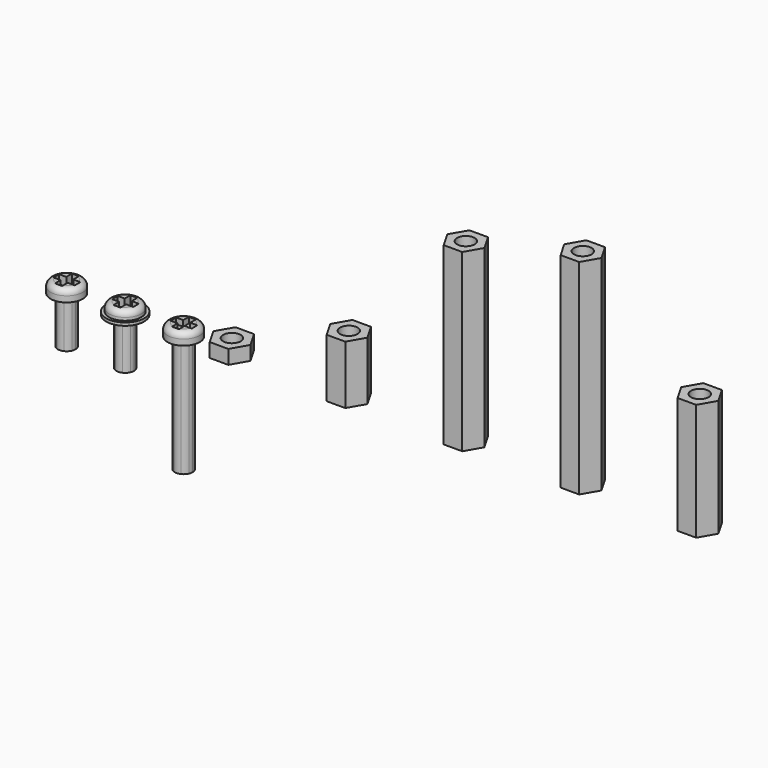
from build123d import *

# Parameters (mm, degrees)
F0_R      = 1.5
F1_DEPTH  = 2.4
F2_DEPTH  = 10
F3_DEPTH  = 30
F4_R      = 2.75
F5_DEPTH  = 2
F6_DEPTH  = 2
F7_DEPTH  = 0.5
F8_DEPTH  = 8
F4_R_2    = 3.25
F12_DEPTH = 0.5
F14_DEPTH = 35
F16_DEPTH = 20
F19_DEPTH = 2
F20_DEPTH = 2
F21_DEPTH = 1
F22_DEPTH = 20


# Not quite as in the source:
# - a fillet or chamfer that OpenCascade refuses, or shapes differently, is made with other operations: its cross-section is extruded or revolved along the edge and cut away or added


with BuildPart() as f1:
    # F0 (on Top) → F1 (new body)
    with BuildSketch(Plane.XY):
        Polygon((1.5877132403, -2.75), (3.1754264805, 0), (1.5877132403, 2.75), (-1.5877132403, 2.75), (-3.1754264805, 0), (-1.5877132403, -2.75), align=None)
        Circle(F0_R, mode=Mode.SUBTRACT)
    extrude(amount=F1_DEPTH)


with BuildPart() as f2:
    # F0 (on Top) → F2 (new body)
    with BuildSketch(Plane.XY):
        Polygon((1.5877132403, -2.75), (3.1754264805, 0), (1.5877132403, 2.75), (-1.5877132403, 2.75), (-3.1754264805, 0), (-1.5877132403, -2.75), align=None)
        Circle(F0_R, mode=Mode.SUBTRACT)
    extrude(amount=F2_DEPTH)


with BuildPart() as f3:
    # F0 (on Top) → F3 (new body)
    with BuildSketch(Plane.XY):
        Polygon((1.5877132403, -2.75), (3.1754264805, 0), (1.5877132403, 2.75), (-1.5877132403, 2.75), (-3.1754264805, 0), (-1.5877132403, -2.75), align=None)
        Circle(F0_R, mode=Mode.SUBTRACT)
    extrude(amount=F3_DEPTH)


with BuildPart() as f5:
    # F4 (on Top) → F5 (new body)
    with BuildSketch(Plane.XY):
        with Locations((-8.2484744489, 0)):
            Circle(F4_R)
        with BuildLine():
            ThreePointArc((-7.6, 1.3525830433), (-7.1691331802, 1.0416440974), (-6.8737017404, 0.6))
            Line((-6.8737017404, 0.6), (-6.4, 0.6))
            Line((-6.4, 0.6), (-6.4, -0.6))
            Line((-6.4, -0.6), (-6.8737017404, -0.6))
            ThreePointArc((-6.8737017404, -0.6), (-7.1691331802, -1.0416440974), (-7.6, -1.3525830433))
            Line((-7.6, -1.3525830433), (-7.6, -1.8))
            Line((-7.6, -1.8), (-8.8, -1.8))
            Line((-8.8, -1.8), (-8.8, -1.394926366))
            ThreePointArc((-8.8, -1.394926366), (-9.2904116966, -1.0790582802), (-9.6232471574, -0.6))
            Line((-9.6232471574, -0.6), (-10, -0.6))
            Line((-10, -0.6), (-10, 0.6))
            Line((-10, 0.6), (-9.6232471574, 0.6))
            ThreePointArc((-9.6232471574, 0.6), (-9.2904116966, 1.0790582802), (-8.8, 1.394926366))
            Line((-8.8, 1.394926366), (-8.8, 1.8))
            Line((-8.8, 1.8), (-7.6, 1.8))
            Line((-7.6, 1.8), (-7.6, 1.3525830433))
        make_face(mode=Mode.SUBTRACT)
        with BuildLine():
            ThreePointArc((-9.6232471574, -0.6), (-9.2904116966, -1.0790582802), (-8.8, -1.394926366))
            Line((-8.8, -1.394926366), (-8.8, -0.6))
            Line((-8.8, -0.6), (-9.6232471574, -0.6))
        make_face()
        with BuildLine():
            ThreePointArc((-9.6232471574, -0.6), (-9.7484744489, 0), (-9.6232471574, 0.6))
            Line((-9.6232471574, 0.6), (-10, 0.6))
            Line((-10, 0.6), (-10, -0.6))
            Line((-10, -0.6), (-9.6232471574, -0.6))
        make_face()
        with BuildLine():
            Line((-7.6, -1.8), (-7.6, -1.3525830433))
            ThreePointArc((-7.6, -1.3525830433), (-8.1955782161, -1.4990670394), (-8.8, -1.394926366))
            Line((-8.8, -1.394926366), (-8.8, -1.8))
            Line((-8.8, -1.8), (-7.6, -1.8))
        make_face()
        with BuildLine():
            ThreePointArc((-7.6, -1.3525830433), (-7.1691331802, -1.0416440974), (-6.8737017404, -0.6))
            Line((-6.8737017404, -0.6), (-7.6, -0.6))
            Line((-7.6, -0.6), (-7.6, -1.3525830433))
        make_face()
        with BuildLine():
            ThreePointArc((-6.8737017404, 0.6), (-6.7801149795, 0.3064644655), (-6.7484744489, 0))
            ThreePointArc((-6.7484744489, 0), (-6.7801149795, -0.3064644655), (-6.8737017404, -0.6))
            Line((-6.8737017404, -0.6), (-6.4, -0.6))
            Line((-6.4, -0.6), (-6.4, 0.6))
            Line((-6.4, 0.6), (-6.8737017404, 0.6))
        make_face()
        with BuildLine():
            Line((-7.6, 0.6), (-6.8737017404, 0.6))
            ThreePointArc((-6.8737017404, 0.6), (-7.1691331802, 1.0416440974), (-7.6, 1.3525830433))
            Line((-7.6, 1.3525830433), (-7.6, 0.6))
        make_face()
        with BuildLine():
            ThreePointArc((-8.8, 1.394926366), (-8.1955782161, 1.4990670394), (-7.6, 1.3525830433))
            Line((-7.6, 1.3525830433), (-7.6, 1.8))
            Line((-7.6, 1.8), (-8.8, 1.8))
            Line((-8.8, 1.8), (-8.8, 1.394926366))
        make_face()
        with BuildLine():
            Line((-8.8, 0.6), (-8.8, 1.394926366))
            ThreePointArc((-8.8, 1.394926366), (-9.2904116966, 1.0790582802), (-9.6232471574, 0.6))
            Line((-9.6232471574, 0.6), (-8.8, 0.6))
        make_face()
        with BuildLine():
            ThreePointArc((-6.8737017404, -0.6), (-6.7801149795, -0.3064644655), (-6.7484744489, 0))
            ThreePointArc((-6.7484744489, 0), (-6.7801149795, 0.3064644655), (-6.8737017404, 0.6))
            Line((-6.8737017404, 0.6), (-7.6, 0.6))
            Line((-7.6, 0.6), (-7.6, 1.3525830433))
            ThreePointArc((-7.6, 1.3525830433), (-8.1955782161, 1.4990670394), (-8.8, 1.394926366))
            Line((-8.8, 1.394926366), (-8.8, 0.6))
            Line((-8.8, 0.6), (-9.6232471574, 0.6))
            ThreePointArc((-9.6232471574, 0.6), (-9.7484744489, 0), (-9.6232471574, -0.6))
            Line((-9.6232471574, -0.6), (-8.8, -0.6))
            Line((-8.8, -0.6), (-8.8, -1.394926366))
            ThreePointArc((-8.8, -1.394926366), (-8.1955782161, -1.4990670394), (-7.6, -1.3525830433))
            Line((-7.6, -1.3525830433), (-7.6, -0.6))
            Line((-7.6, -0.6), (-6.8737017404, -0.6))
        make_face()
    extrude(amount=F5_DEPTH)

    # F4 (on Top) → F6 (cut)
    with BuildSketch(Plane.XY):
        with BuildLine():
            ThreePointArc((-9.6232471574, -0.6), (-9.7484744489, 0), (-9.6232471574, 0.6))
            Line((-9.6232471574, 0.6), (-10, 0.6))
            Line((-10, 0.6), (-10, -0.6))
            Line((-10, -0.6), (-9.6232471574, -0.6))
        make_face()
        with BuildLine():
            ThreePointArc((-6.8737017404, -0.6), (-6.7801149795, -0.3064644655), (-6.7484744489, 0))
            ThreePointArc((-6.7484744489, 0), (-6.7801149795, 0.3064644655), (-6.8737017404, 0.6))
            Line((-6.8737017404, 0.6), (-7.6, 0.6))
            Line((-7.6, 0.6), (-7.6, 1.3525830433))
            ThreePointArc((-7.6, 1.3525830433), (-8.1955782161, 1.4990670394), (-8.8, 1.394926366))
            Line((-8.8, 1.394926366), (-8.8, 0.6))
            Line((-8.8, 0.6), (-9.6232471574, 0.6))
            ThreePointArc((-9.6232471574, 0.6), (-9.7484744489, 0), (-9.6232471574, -0.6))
            Line((-9.6232471574, -0.6), (-8.8, -0.6))
            Line((-8.8, -0.6), (-8.8, -1.394926366))
            ThreePointArc((-8.8, -1.394926366), (-8.1955782161, -1.4990670394), (-7.6, -1.3525830433))
            Line((-7.6, -1.3525830433), (-7.6, -0.6))
            Line((-7.6, -0.6), (-6.8737017404, -0.6))
        make_face()
        with BuildLine():
            ThreePointArc((-6.8737017404, 0.6), (-6.7801149795, 0.3064644655), (-6.7484744489, 0))
            ThreePointArc((-6.7484744489, 0), (-6.7801149795, -0.3064644655), (-6.8737017404, -0.6))
            Line((-6.8737017404, -0.6), (-6.4, -0.6))
            Line((-6.4, -0.6), (-6.4, 0.6))
            Line((-6.4, 0.6), (-6.8737017404, 0.6))
        make_face()
        with BuildLine():
            Line((-7.6, -1.8), (-7.6, -1.3525830433))
            ThreePointArc((-7.6, -1.3525830433), (-8.1955782161, -1.4990670394), (-8.8, -1.394926366))
            Line((-8.8, -1.394926366), (-8.8, -1.8))
            Line((-8.8, -1.8), (-7.6, -1.8))
        make_face()
        with BuildLine():
            ThreePointArc((-8.8, 1.394926366), (-8.1955782161, 1.4990670394), (-7.6, 1.3525830433))
            Line((-7.6, 1.3525830433), (-7.6, 1.8))
            Line((-7.6, 1.8), (-8.8, 1.8))
            Line((-8.8, 1.8), (-8.8, 1.394926366))
        make_face()
    extrude(amount=F6_DEPTH, mode=Mode.SUBTRACT)

    # F4 (on Top) → F7 (join)
    with BuildSketch(Plane.XY):
        with Locations((-8.2484744489, 0)):
            Circle(F4_R)
        with BuildLine():
            ThreePointArc((-7.6, 1.3525830433), (-7.1691331802, 1.0416440974), (-6.8737017404, 0.6))
            Line((-6.8737017404, 0.6), (-6.4, 0.6))
            Line((-6.4, 0.6), (-6.4, -0.6))
            Line((-6.4, -0.6), (-6.8737017404, -0.6))
            ThreePointArc((-6.8737017404, -0.6), (-7.1691331802, -1.0416440974), (-7.6, -1.3525830433))
            Line((-7.6, -1.3525830433), (-7.6, -1.8))
            Line((-7.6, -1.8), (-8.8, -1.8))
            Line((-8.8, -1.8), (-8.8, -1.394926366))
            ThreePointArc((-8.8, -1.394926366), (-9.2904116966, -1.0790582802), (-9.6232471574, -0.6))
            Line((-9.6232471574, -0.6), (-10, -0.6))
            Line((-10, -0.6), (-10, 0.6))
            Line((-10, 0.6), (-9.6232471574, 0.6))
            ThreePointArc((-9.6232471574, 0.6), (-9.2904116966, 1.0790582802), (-8.8, 1.394926366))
            Line((-8.8, 1.394926366), (-8.8, 1.8))
            Line((-8.8, 1.8), (-7.6, 1.8))
            Line((-7.6, 1.8), (-7.6, 1.3525830433))
        make_face(mode=Mode.SUBTRACT)
        with BuildLine():
            ThreePointArc((-9.6232471574, -0.6), (-9.2904116966, -1.0790582802), (-8.8, -1.394926366))
            Line((-8.8, -1.394926366), (-8.8, -0.6))
            Line((-8.8, -0.6), (-9.6232471574, -0.6))
        make_face()
        with BuildLine():
            Line((-7.6, -1.8), (-7.6, -1.3525830433))
            ThreePointArc((-7.6, -1.3525830433), (-8.1955782161, -1.4990670394), (-8.8, -1.394926366))
            Line((-8.8, -1.394926366), (-8.8, -1.8))
            Line((-8.8, -1.8), (-7.6, -1.8))
        make_face()
        with BuildLine():
            ThreePointArc((-7.6, -1.3525830433), (-7.1691331802, -1.0416440974), (-6.8737017404, -0.6))
            Line((-6.8737017404, -0.6), (-7.6, -0.6))
            Line((-7.6, -0.6), (-7.6, -1.3525830433))
        make_face()
        with BuildLine():
            ThreePointArc((-6.8737017404, 0.6), (-6.7801149795, 0.3064644655), (-6.7484744489, 0))
            ThreePointArc((-6.7484744489, 0), (-6.7801149795, -0.3064644655), (-6.8737017404, -0.6))
            Line((-6.8737017404, -0.6), (-6.4, -0.6))
            Line((-6.4, -0.6), (-6.4, 0.6))
            Line((-6.4, 0.6), (-6.8737017404, 0.6))
        make_face()
        with BuildLine():
            ThreePointArc((-6.8737017404, -0.6), (-6.7801149795, -0.3064644655), (-6.7484744489, 0))
            ThreePointArc((-6.7484744489, 0), (-6.7801149795, 0.3064644655), (-6.8737017404, 0.6))
            Line((-6.8737017404, 0.6), (-7.6, 0.6))
            Line((-7.6, 0.6), (-7.6, 1.3525830433))
            ThreePointArc((-7.6, 1.3525830433), (-8.1955782161, 1.4990670394), (-8.8, 1.394926366))
            Line((-8.8, 1.394926366), (-8.8, 0.6))
            Line((-8.8, 0.6), (-9.6232471574, 0.6))
            ThreePointArc((-9.6232471574, 0.6), (-9.7484744489, 0), (-9.6232471574, -0.6))
            Line((-9.6232471574, -0.6), (-8.8, -0.6))
            Line((-8.8, -0.6), (-8.8, -1.394926366))
            ThreePointArc((-8.8, -1.394926366), (-8.1955782161, -1.4990670394), (-7.6, -1.3525830433))
            Line((-7.6, -1.3525830433), (-7.6, -0.6))
            Line((-7.6, -0.6), (-6.8737017404, -0.6))
        make_face()
        with BuildLine():
            ThreePointArc((-8.8, 1.394926366), (-8.1955782161, 1.4990670394), (-7.6, 1.3525830433))
            Line((-7.6, 1.3525830433), (-7.6, 1.8))
            Line((-7.6, 1.8), (-8.8, 1.8))
            Line((-8.8, 1.8), (-8.8, 1.394926366))
        make_face()
        with BuildLine():
            Line((-8.8, 0.6), (-8.8, 1.394926366))
            ThreePointArc((-8.8, 1.394926366), (-9.2904116966, 1.0790582802), (-9.6232471574, 0.6))
            Line((-9.6232471574, 0.6), (-8.8, 0.6))
        make_face()
        with BuildLine():
            Line((-7.6, 0.6), (-6.8737017404, 0.6))
            ThreePointArc((-6.8737017404, 0.6), (-7.1691331802, 1.0416440974), (-7.6, 1.3525830433))
            Line((-7.6, 1.3525830433), (-7.6, 0.6))
        make_face()
        with BuildLine():
            ThreePointArc((-9.6232471574, -0.6), (-9.7484744489, 0), (-9.6232471574, 0.6))
            Line((-9.6232471574, 0.6), (-10, 0.6))
            Line((-10, 0.6), (-10, -0.6))
            Line((-10, -0.6), (-9.6232471574, -0.6))
        make_face()
    extrude(amount=F7_DEPTH)

    # F4 (on Top) → F8 (join)
    with BuildSketch(Plane.XY):
        with BuildLine():
            ThreePointArc((-9.6232471574, -0.6), (-9.2904116966, -1.0790582802), (-8.8, -1.394926366))
            Line((-8.8, -1.394926366), (-8.8, -0.6))
            Line((-8.8, -0.6), (-9.6232471574, -0.6))
        make_face()
        with BuildLine():
            ThreePointArc((-6.8737017404, -0.6), (-6.7801149795, -0.3064644655), (-6.7484744489, 0))
            ThreePointArc((-6.7484744489, 0), (-6.7801149795, 0.3064644655), (-6.8737017404, 0.6))
            Line((-6.8737017404, 0.6), (-7.6, 0.6))
            Line((-7.6, 0.6), (-7.6, 1.3525830433))
            ThreePointArc((-7.6, 1.3525830433), (-8.1955782161, 1.4990670394), (-8.8, 1.394926366))
            Line((-8.8, 1.394926366), (-8.8, 0.6))
            Line((-8.8, 0.6), (-9.6232471574, 0.6))
            ThreePointArc((-9.6232471574, 0.6), (-9.7484744489, 0), (-9.6232471574, -0.6))
            Line((-9.6232471574, -0.6), (-8.8, -0.6))
            Line((-8.8, -0.6), (-8.8, -1.394926366))
            ThreePointArc((-8.8, -1.394926366), (-8.1955782161, -1.4990670394), (-7.6, -1.3525830433))
            Line((-7.6, -1.3525830433), (-7.6, -0.6))
            Line((-7.6, -0.6), (-6.8737017404, -0.6))
        make_face()
        with BuildLine():
            ThreePointArc((-7.6, -1.3525830433), (-7.1691331802, -1.0416440974), (-6.8737017404, -0.6))
            Line((-6.8737017404, -0.6), (-7.6, -0.6))
            Line((-7.6, -0.6), (-7.6, -1.3525830433))
        make_face()
        with BuildLine():
            Line((-8.8, 0.6), (-8.8, 1.394926366))
            ThreePointArc((-8.8, 1.394926366), (-9.2904116966, 1.0790582802), (-9.6232471574, 0.6))
            Line((-9.6232471574, 0.6), (-8.8, 0.6))
        make_face()
        with BuildLine():
            Line((-7.6, 0.6), (-6.8737017404, 0.6))
            ThreePointArc((-6.8737017404, 0.6), (-7.1691331802, 1.0416440974), (-7.6, 1.3525830433))
            Line((-7.6, 1.3525830433), (-7.6, 0.6))
        make_face()
    extrude(amount=-F8_DEPTH)


with BuildPart() as f2_1:
    # F9: moved
    add(f2.part.moved(Location((20, 0, 0))))


with BuildPart() as f3_1:
    # F10: moved
    add(f3.part.moved(Location((40, 0, 0))))


with BuildPart() as f11_1:
    # F11: copy of F5
    add(f5.part.moved(Location((-20, 0, 0))))

    # F13: fillet of radius 1 on 1 edges, made by hand

    # F13_s1 → F13_t2 (revolve, cut)
    with BuildSketch(Plane.XZ):
        with BuildLine():
            ThreePointArc((-25.4984744489, 1), (-25.7913676677, 1.7071067812), (-26.4984744489, 2))
            Line((-26.4984744489, 2), (-25.4984744489, 2))
            Line((-25.4984744489, 2), (-25.4984744489, 1))
        make_face()
    revolve(axis=Axis((-28.2484744489, 0, 2), (0, 0, 1)), mode=Mode.SUBTRACT)


with BuildPart() as f5_1:
    add(f5.part)

    # F4 (on Top) → F12 (join)
    with BuildSketch(Plane.XY):
        with Locations((-8.2484744489, 0)):
            Circle(F4_R_2)
        with Locations((-8.2484744489, 0)):
            Circle(F4_R, mode=Mode.SUBTRACT)
    extrude(amount=F12_DEPTH)

    # F13#2: fillet of radius 1 on 1 edges, made by hand

    # F13_2_s1 → F13_2_t2 (revolve, cut)
    with BuildSketch(Plane.XZ):
        with BuildLine():
            ThreePointArc((-5.4984744489, 1), (-5.7913676677, 1.7071067812), (-6.4984744489, 2))
            Line((-6.4984744489, 2), (-5.4984744489, 2))
            Line((-5.4984744489, 2), (-5.4984744489, 1))
        make_face()
    revolve(axis=Axis((-8.2484744489, 0, 2), (0, 0, 1)), mode=Mode.SUBTRACT)


with BuildPart() as f14:
    # F0 (on Top) → F14 (new body)
    with BuildSketch(Plane.XY):
        Polygon((1.5877132403, -2.75), (3.1754264805, 0), (1.5877132403, 2.75), (-1.5877132403, 2.75), (-3.1754264805, 0), (-1.5877132403, -2.75), align=None)
        Circle(F0_R, mode=Mode.SUBTRACT)
    extrude(amount=F14_DEPTH)


with BuildPart() as f14_1:
    # F15: moved
    add(f14.part.moved(Location((60, 0, 0))))


with BuildPart() as f16:
    # F0 (on Top) → F16 (new body)
    with BuildSketch(Plane.XY):
        Polygon((1.5877132403, -2.75), (3.1754264805, 0), (1.5877132403, 2.75), (-1.5877132403, 2.75), (-3.1754264805, 0), (-1.5877132403, -2.75), align=None)
        Circle(F0_R, mode=Mode.SUBTRACT)
    extrude(amount=F16_DEPTH)


with BuildPart() as f16_1:
    # F17: moved
    add(f16.part.moved(Location((80, 0, 0))))


with BuildPart() as f5_2:
    # F18: moved
    add(f5_1.part.moved(Location((-10, 0, 0))))


with BuildPart() as f19:
    # F4 (on Top) → F19 (new body)
    with BuildSketch(Plane.XY):
        with Locations((-8.2484744489, 0)):
            Circle(F4_R)
        with BuildLine():
            ThreePointArc((-7.6, 1.3525830433), (-7.1691331802, 1.0416440974), (-6.8737017404, 0.6))
            Line((-6.8737017404, 0.6), (-6.4, 0.6))
            Line((-6.4, 0.6), (-6.4, -0.6))
            Line((-6.4, -0.6), (-6.8737017404, -0.6))
            ThreePointArc((-6.8737017404, -0.6), (-7.1691331802, -1.0416440974), (-7.6, -1.3525830433))
            Line((-7.6, -1.3525830433), (-7.6, -1.8))
            Line((-7.6, -1.8), (-8.8, -1.8))
            Line((-8.8, -1.8), (-8.8, -1.394926366))
            ThreePointArc((-8.8, -1.394926366), (-9.2904116966, -1.0790582802), (-9.6232471574, -0.6))
            Line((-9.6232471574, -0.6), (-10, -0.6))
            Line((-10, -0.6), (-10, 0.6))
            Line((-10, 0.6), (-9.6232471574, 0.6))
            ThreePointArc((-9.6232471574, 0.6), (-9.2904116966, 1.0790582802), (-8.8, 1.394926366))
            Line((-8.8, 1.394926366), (-8.8, 1.8))
            Line((-8.8, 1.8), (-7.6, 1.8))
            Line((-7.6, 1.8), (-7.6, 1.3525830433))
        make_face(mode=Mode.SUBTRACT)
        with BuildLine():
            ThreePointArc((-6.8737017404, 0.6), (-6.7801149795, 0.3064644655), (-6.7484744489, 0))
            ThreePointArc((-6.7484744489, 0), (-6.7801149795, -0.3064644655), (-6.8737017404, -0.6))
            Line((-6.8737017404, -0.6), (-6.4, -0.6))
            Line((-6.4, -0.6), (-6.4, 0.6))
            Line((-6.4, 0.6), (-6.8737017404, 0.6))
        make_face()
        with BuildLine():
            ThreePointArc((-7.6, -1.3525830433), (-7.1691331802, -1.0416440974), (-6.8737017404, -0.6))
            Line((-6.8737017404, -0.6), (-7.6, -0.6))
            Line((-7.6, -0.6), (-7.6, -1.3525830433))
        make_face()
        with BuildLine():
            ThreePointArc((-9.6232471574, -0.6), (-9.2904116966, -1.0790582802), (-8.8, -1.394926366))
            Line((-8.8, -1.394926366), (-8.8, -0.6))
            Line((-8.8, -0.6), (-9.6232471574, -0.6))
        make_face()
        with BuildLine():
            Line((-7.6, -1.8), (-7.6, -1.3525830433))
            ThreePointArc((-7.6, -1.3525830433), (-8.1955782161, -1.4990670394), (-8.8, -1.394926366))
            Line((-8.8, -1.394926366), (-8.8, -1.8))
            Line((-8.8, -1.8), (-7.6, -1.8))
        make_face()
        with BuildLine():
            ThreePointArc((-9.6232471574, -0.6), (-9.7484744489, 0), (-9.6232471574, 0.6))
            Line((-9.6232471574, 0.6), (-10, 0.6))
            Line((-10, 0.6), (-10, -0.6))
            Line((-10, -0.6), (-9.6232471574, -0.6))
        make_face()
        with BuildLine():
            ThreePointArc((-8.8, 1.394926366), (-8.1955782161, 1.4990670394), (-7.6, 1.3525830433))
            Line((-7.6, 1.3525830433), (-7.6, 1.8))
            Line((-7.6, 1.8), (-8.8, 1.8))
            Line((-8.8, 1.8), (-8.8, 1.394926366))
        make_face()
        with BuildLine():
            Line((-7.6, 0.6), (-6.8737017404, 0.6))
            ThreePointArc((-6.8737017404, 0.6), (-7.1691331802, 1.0416440974), (-7.6, 1.3525830433))
            Line((-7.6, 1.3525830433), (-7.6, 0.6))
        make_face()
        with BuildLine():
            Line((-8.8, 0.6), (-8.8, 1.394926366))
            ThreePointArc((-8.8, 1.394926366), (-9.2904116966, 1.0790582802), (-9.6232471574, 0.6))
            Line((-9.6232471574, 0.6), (-8.8, 0.6))
        make_face()
        with BuildLine():
            ThreePointArc((-6.8737017404, -0.6), (-6.7801149795, -0.3064644655), (-6.7484744489, 0))
            ThreePointArc((-6.7484744489, 0), (-6.7801149795, 0.3064644655), (-6.8737017404, 0.6))
            Line((-6.8737017404, 0.6), (-7.6, 0.6))
            Line((-7.6, 0.6), (-7.6, 1.3525830433))
            ThreePointArc((-7.6, 1.3525830433), (-8.1955782161, 1.4990670394), (-8.8, 1.394926366))
            Line((-8.8, 1.394926366), (-8.8, 0.6))
            Line((-8.8, 0.6), (-9.6232471574, 0.6))
            ThreePointArc((-9.6232471574, 0.6), (-9.7484744489, 0), (-9.6232471574, -0.6))
            Line((-9.6232471574, -0.6), (-8.8, -0.6))
            Line((-8.8, -0.6), (-8.8, -1.394926366))
            ThreePointArc((-8.8, -1.394926366), (-8.1955782161, -1.4990670394), (-7.6, -1.3525830433))
            Line((-7.6, -1.3525830433), (-7.6, -0.6))
            Line((-7.6, -0.6), (-6.8737017404, -0.6))
        make_face()
    extrude(amount=F19_DEPTH)

    # F4 (on Top) → F20 (cut)
    with BuildSketch(Plane.XY):
        with BuildLine():
            ThreePointArc((-6.8737017404, -0.6), (-6.7801149795, -0.3064644655), (-6.7484744489, 0))
            ThreePointArc((-6.7484744489, 0), (-6.7801149795, 0.3064644655), (-6.8737017404, 0.6))
            Line((-6.8737017404, 0.6), (-7.6, 0.6))
            Line((-7.6, 0.6), (-7.6, 1.3525830433))
            ThreePointArc((-7.6, 1.3525830433), (-8.1955782161, 1.4990670394), (-8.8, 1.394926366))
            Line((-8.8, 1.394926366), (-8.8, 0.6))
            Line((-8.8, 0.6), (-9.6232471574, 0.6))
            ThreePointArc((-9.6232471574, 0.6), (-9.7484744489, 0), (-9.6232471574, -0.6))
            Line((-9.6232471574, -0.6), (-8.8, -0.6))
            Line((-8.8, -0.6), (-8.8, -1.394926366))
            ThreePointArc((-8.8, -1.394926366), (-8.1955782161, -1.4990670394), (-7.6, -1.3525830433))
            Line((-7.6, -1.3525830433), (-7.6, -0.6))
            Line((-7.6, -0.6), (-6.8737017404, -0.6))
        make_face()
        with BuildLine():
            Line((-7.6, -1.8), (-7.6, -1.3525830433))
            ThreePointArc((-7.6, -1.3525830433), (-8.1955782161, -1.4990670394), (-8.8, -1.394926366))
            Line((-8.8, -1.394926366), (-8.8, -1.8))
            Line((-8.8, -1.8), (-7.6, -1.8))
        make_face()
        with BuildLine():
            ThreePointArc((-9.6232471574, -0.6), (-9.7484744489, 0), (-9.6232471574, 0.6))
            Line((-9.6232471574, 0.6), (-10, 0.6))
            Line((-10, 0.6), (-10, -0.6))
            Line((-10, -0.6), (-9.6232471574, -0.6))
        make_face()
        with BuildLine():
            ThreePointArc((-8.8, 1.394926366), (-8.1955782161, 1.4990670394), (-7.6, 1.3525830433))
            Line((-7.6, 1.3525830433), (-7.6, 1.8))
            Line((-7.6, 1.8), (-8.8, 1.8))
            Line((-8.8, 1.8), (-8.8, 1.394926366))
        make_face()
        with BuildLine():
            ThreePointArc((-6.8737017404, 0.6), (-6.7801149795, 0.3064644655), (-6.7484744489, 0))
            ThreePointArc((-6.7484744489, 0), (-6.7801149795, -0.3064644655), (-6.8737017404, -0.6))
            Line((-6.8737017404, -0.6), (-6.4, -0.6))
            Line((-6.4, -0.6), (-6.4, 0.6))
            Line((-6.4, 0.6), (-6.8737017404, 0.6))
        make_face()
    extrude(amount=F20_DEPTH, mode=Mode.SUBTRACT)

    # F4 (on Top) → F21 (join)
    with BuildSketch(Plane.XY):
        with Locations((-8.2484744489, 0)):
            Circle(F4_R)
        with BuildLine():
            ThreePointArc((-7.6, 1.3525830433), (-7.1691331802, 1.0416440974), (-6.8737017404, 0.6))
            Line((-6.8737017404, 0.6), (-6.4, 0.6))
            Line((-6.4, 0.6), (-6.4, -0.6))
            Line((-6.4, -0.6), (-6.8737017404, -0.6))
            ThreePointArc((-6.8737017404, -0.6), (-7.1691331802, -1.0416440974), (-7.6, -1.3525830433))
            Line((-7.6, -1.3525830433), (-7.6, -1.8))
            Line((-7.6, -1.8), (-8.8, -1.8))
            Line((-8.8, -1.8), (-8.8, -1.394926366))
            ThreePointArc((-8.8, -1.394926366), (-9.2904116966, -1.0790582802), (-9.6232471574, -0.6))
            Line((-9.6232471574, -0.6), (-10, -0.6))
            Line((-10, -0.6), (-10, 0.6))
            Line((-10, 0.6), (-9.6232471574, 0.6))
            ThreePointArc((-9.6232471574, 0.6), (-9.2904116966, 1.0790582802), (-8.8, 1.394926366))
            Line((-8.8, 1.394926366), (-8.8, 1.8))
            Line((-8.8, 1.8), (-7.6, 1.8))
            Line((-7.6, 1.8), (-7.6, 1.3525830433))
        make_face(mode=Mode.SUBTRACT)
        with BuildLine():
            Line((-7.6, -1.8), (-7.6, -1.3525830433))
            ThreePointArc((-7.6, -1.3525830433), (-8.1955782161, -1.4990670394), (-8.8, -1.394926366))
            Line((-8.8, -1.394926366), (-8.8, -1.8))
            Line((-8.8, -1.8), (-7.6, -1.8))
        make_face()
        with BuildLine():
            ThreePointArc((-6.8737017404, 0.6), (-6.7801149795, 0.3064644655), (-6.7484744489, 0))
            ThreePointArc((-6.7484744489, 0), (-6.7801149795, -0.3064644655), (-6.8737017404, -0.6))
            Line((-6.8737017404, -0.6), (-6.4, -0.6))
            Line((-6.4, -0.6), (-6.4, 0.6))
            Line((-6.4, 0.6), (-6.8737017404, 0.6))
        make_face()
        with BuildLine():
            ThreePointArc((-9.6232471574, -0.6), (-9.7484744489, 0), (-9.6232471574, 0.6))
            Line((-9.6232471574, 0.6), (-10, 0.6))
            Line((-10, 0.6), (-10, -0.6))
            Line((-10, -0.6), (-9.6232471574, -0.6))
        make_face()
        with BuildLine():
            ThreePointArc((-8.8, 1.394926366), (-8.1955782161, 1.4990670394), (-7.6, 1.3525830433))
            Line((-7.6, 1.3525830433), (-7.6, 1.8))
            Line((-7.6, 1.8), (-8.8, 1.8))
            Line((-8.8, 1.8), (-8.8, 1.394926366))
        make_face()
        with BuildLine():
            ThreePointArc((-6.8737017404, -0.6), (-6.7801149795, -0.3064644655), (-6.7484744489, 0))
            ThreePointArc((-6.7484744489, 0), (-6.7801149795, 0.3064644655), (-6.8737017404, 0.6))
            Line((-6.8737017404, 0.6), (-7.6, 0.6))
            Line((-7.6, 0.6), (-7.6, 1.3525830433))
            ThreePointArc((-7.6, 1.3525830433), (-8.1955782161, 1.4990670394), (-8.8, 1.394926366))
            Line((-8.8, 1.394926366), (-8.8, 0.6))
            Line((-8.8, 0.6), (-9.6232471574, 0.6))
            ThreePointArc((-9.6232471574, 0.6), (-9.7484744489, 0), (-9.6232471574, -0.6))
            Line((-9.6232471574, -0.6), (-8.8, -0.6))
            Line((-8.8, -0.6), (-8.8, -1.394926366))
            ThreePointArc((-8.8, -1.394926366), (-8.1955782161, -1.4990670394), (-7.6, -1.3525830433))
            Line((-7.6, -1.3525830433), (-7.6, -0.6))
            Line((-7.6, -0.6), (-6.8737017404, -0.6))
        make_face()
    extrude(amount=F21_DEPTH)

    # F4 (on Top) → F22 (join)
    with BuildSketch(Plane.XY):
        with BuildLine():
            ThreePointArc((-9.6232471574, -0.6), (-9.2904116966, -1.0790582802), (-8.8, -1.394926366))
            Line((-8.8, -1.394926366), (-8.8, -0.6))
            Line((-8.8, -0.6), (-9.6232471574, -0.6))
        make_face()
        with BuildLine():
            ThreePointArc((-6.8737017404, -0.6), (-6.7801149795, -0.3064644655), (-6.7484744489, 0))
            ThreePointArc((-6.7484744489, 0), (-6.7801149795, 0.3064644655), (-6.8737017404, 0.6))
            Line((-6.8737017404, 0.6), (-7.6, 0.6))
            Line((-7.6, 0.6), (-7.6, 1.3525830433))
            ThreePointArc((-7.6, 1.3525830433), (-8.1955782161, 1.4990670394), (-8.8, 1.394926366))
            Line((-8.8, 1.394926366), (-8.8, 0.6))
            Line((-8.8, 0.6), (-9.6232471574, 0.6))
            ThreePointArc((-9.6232471574, 0.6), (-9.7484744489, 0), (-9.6232471574, -0.6))
            Line((-9.6232471574, -0.6), (-8.8, -0.6))
            Line((-8.8, -0.6), (-8.8, -1.394926366))
            ThreePointArc((-8.8, -1.394926366), (-8.1955782161, -1.4990670394), (-7.6, -1.3525830433))
            Line((-7.6, -1.3525830433), (-7.6, -0.6))
            Line((-7.6, -0.6), (-6.8737017404, -0.6))
        make_face()
        with BuildLine():
            ThreePointArc((-7.6, -1.3525830433), (-7.1691331802, -1.0416440974), (-6.8737017404, -0.6))
            Line((-6.8737017404, -0.6), (-7.6, -0.6))
            Line((-7.6, -0.6), (-7.6, -1.3525830433))
        make_face()
        with BuildLine():
            Line((-7.6, 0.6), (-6.8737017404, 0.6))
            ThreePointArc((-6.8737017404, 0.6), (-7.1691331802, 1.0416440974), (-7.6, 1.3525830433))
            Line((-7.6, 1.3525830433), (-7.6, 0.6))
        make_face()
        with BuildLine():
            Line((-8.8, 0.6), (-8.8, 1.394926366))
            ThreePointArc((-8.8, 1.394926366), (-9.2904116966, 1.0790582802), (-9.6232471574, 0.6))
            Line((-9.6232471574, 0.6), (-8.8, 0.6))
        make_face()
    extrude(amount=-F22_DEPTH)

    # F23: fillet of radius 1 on 1 edges, made by hand

    # F23_s1 → F23_t2 (revolve, cut)
    with BuildSketch(Plane.XZ):
        with BuildLine():
            ThreePointArc((-5.4984744489, 1), (-5.7913676677, 1.7071067812), (-6.4984744489, 2))
            Line((-6.4984744489, 2), (-5.4984744489, 2))
            Line((-5.4984744489, 2), (-5.4984744489, 1))
        make_face()
    revolve(axis=Axis((-8.2484744489, 0, 2), (0, 0, 1)), mode=Mode.SUBTRACT)


solid = Compound([f1.part, f2_1.part, f3_1.part, f11_1.part, f14_1.part, f16_1.part, f5_2.part, f19.part])
